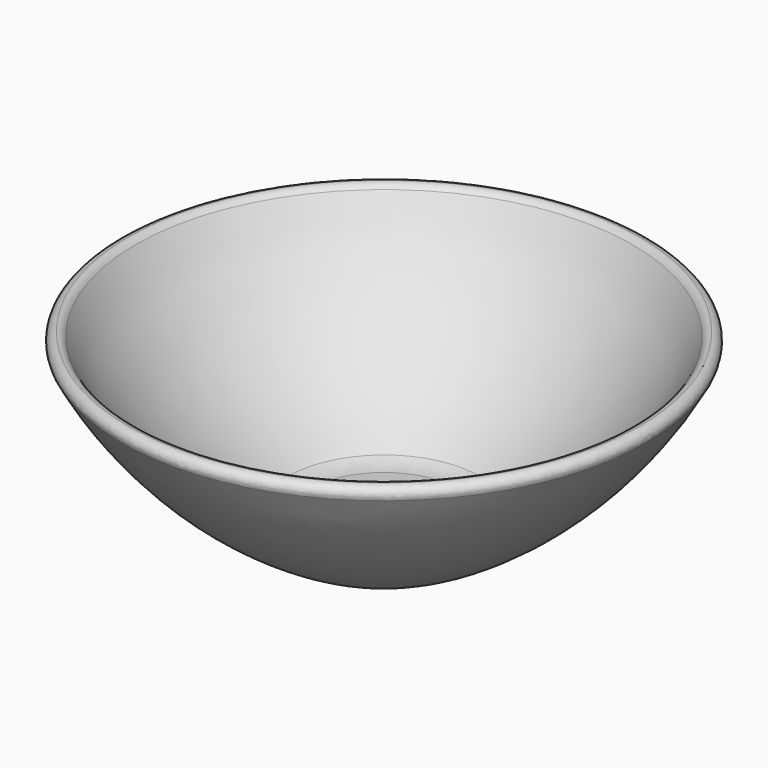
from build123d import *

# Parameters (mm, degrees)
F2_T = -2
F3_R = 0.999
F4_R = 5


# Not quite as in the source:
# - a fillet or chamfer is up to 0.001 mm smaller than in the source, because OpenCascade refuses the exact size


with BuildPart() as f1:
    # F0 (on Front) → F1 (revolve)
    with BuildSketch(Plane.XZ):
        with BuildLine():
            Line((0, 0), (11, 0))
            ThreePointArc((11, 0), (23.7547438265, 9.2452561735), (33, 22))
            Line((33, 22), (0, 22))
            Line((0, 22), (0, 0))
        make_face()
    revolve(axis=Axis((0, 0, 0.8752791786), (0, 0, 1)))

    # F2
    f2_openings = [f1.faces().sort_by_distance(p)[0] for p in [
        (0, 0, 22),
    ]]
    offset(amount=F2_T, openings=f2_openings)

    # F3 (radius 1 in the source; OpenCascade refuses exactly that, so slightly less here)
    f3_edges = [f1.edges().sort_by_distance(p)[0] for p in [
        (-33, 0, 22),
        (-30.745752, 0, 22),
    ]]
    fillet(f3_edges, radius=F3_R)

    # F4
    f4_edges = [f1.edges().sort_by_distance(p)[0] for p in [
        (-10.517029, 0, 2),
    ]]
    fillet(f4_edges, radius=F4_R)


solid = f1.part
